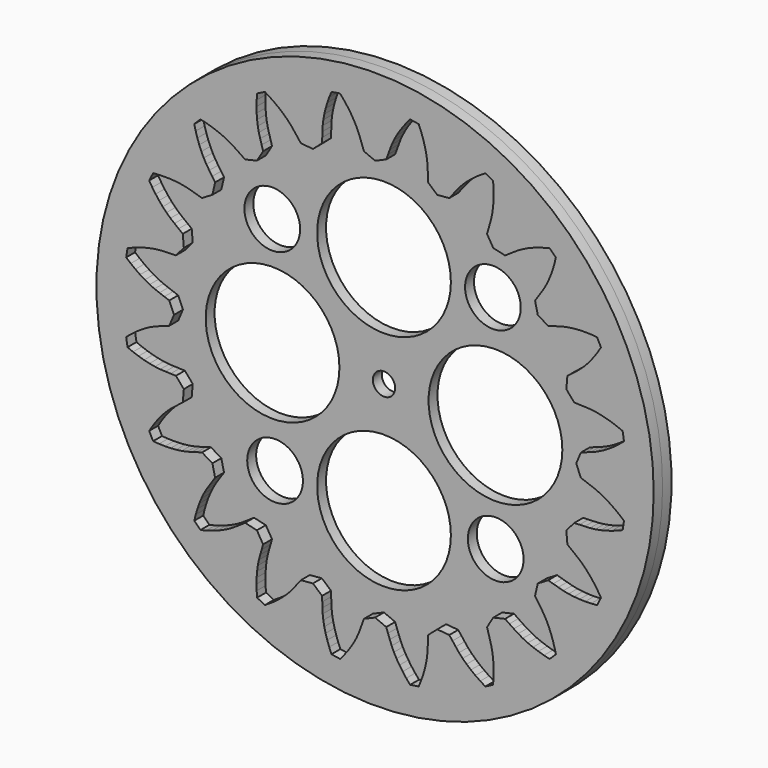
from build123d import *

# Parameters (mm, degrees)
F0_R     = 125
F1_DEPTH = 5
F2_R     = 125
F3_DEPTH = 5
F4_R     = 5
F5_DEPTH = 10.001
F6_R     = 30
F7_DEPTH = 5.001
F8_R     = 12.5
F9_DEPTH = 10.001


# Not quite as in the source:
# - ends of sketch curves that miss each other by under 0.0002 mm in the source are joined


with BuildPart() as f1:
    # F0 (on Front) → F1 (new body)
    with BuildSketch(Plane.XZ):
        Circle(F0_R)
        Polygon((13.9842229545, 109.6228580511), (15.7057802544, 111.6674669584), (19.5700724052, 111.0554232512), (20.5755500849, 108.5788944008), (21.4485215555, 106.1098402186), (22.1849061713, 103.653016947), (22.779065605, 101.2135667406), (23.2227934587, 98.7972702634), (23.5031701941, 96.4110969894), (23.6169992555, 94.0596036896), (23.6990010858, 91.7113680901), (23.7811743213, 89.3582248904), (27.8774327783, 85.7978872065), (33.2840906682, 86.2705394296), (34.7337131873, 88.1259711729), (36.1803125604, 89.9775337706), (37.6545753224, 91.8130253807), (39.2839627575, 93.57867791), (41.0632104221, 95.2726860912), (42.9777689252, 96.8970045446), (45.0176015427, 98.4517796161), (47.1751233459, 99.9361663084), (49.4442399292, 101.3487141929), (52.930256939, 99.572499698), (53.1212343584, 96.9064699183), (53.1884993548, 94.2884977338), (53.1296422324, 91.7243648109), (52.9408900729, 89.2207038275), (52.6162246508, 86.785549776), (52.1455100076, 84.4295237621), (51.5271162906, 82.1579453597), (50.8794594033, 79.8993005287), (50.2304503198, 77.6359355406), (53.0260192955, 72.9840387035), (58.3141129314, 71.7628090439), (60.2661460143, 73.0794722829), (62.2141084754, 74.3933890299), (64.1834143867, 75.6834724412), (66.2786700093, 76.8592005473), (68.4943121935, 77.9204791254), (70.8171076594, 78.8736672065), (73.2375549479, 79.7220024436), (75.7481813959, 80.4670274831), (78.3427412398, 81.1092455143), (81.1092595475, 78.3427262043), (80.4670415162, 75.7481663603), (79.7220164768, 73.2375409148), (78.8736802373, 70.8170926238), (77.9204921562, 68.4942981603), (76.8592125757, 66.2786559761), (75.6834844697, 64.1834003535), (74.3934000559, 62.2140944422), (73.0794833089, 60.2661329835), (71.76282007, 58.3140999006), (72.9840487272, 53.0260052624), (77.6359445619, 50.2304352843), (79.8993095501, 50.8794453702), (82.157954381, 51.5271002527), (84.4295327834, 52.1454939697), (86.7855597997, 52.6162076106), (89.2207138511, 52.9408730326), (91.7243748346, 53.1296251921), (94.2885077575, 53.1884813122), (96.9064799419, 53.1212163158), (99.5725097217, 52.930237894), (101.3487232143, 49.4442208842), (99.9361753297, 47.1751043009), (98.4517876351, 45.0175824977), (96.8970125636, 42.9777508825), (95.2726931078, 41.0631923794), (93.5786859289, 39.2839457173), (91.8130323973, 37.6545582821), (89.9775407871, 36.1802955202), (88.1259771871, 34.733696147), (86.2705454438, 33.2840746303), (85.7978922183, 27.8774167404), (89.3582299022, 23.7811572811), (91.7113720996, 23.6989840456), (94.0596076991, 23.6169812128), (96.4111020013, 23.5031521515), (98.7972742729, 23.222775416), (101.2135707501, 22.7790465599), (103.6530219588, 22.1848861239), (106.1098442281, 21.4485015081), (108.5788974079, 20.5755300376), (111.0554272607, 19.5700513555), (111.6674689632, 15.7057712331), (109.6228590534, 13.9842149355), (107.5444121621, 12.3909899788), (105.4353899991, 10.9314470105), (103.298940004, 9.6125364595), (101.1380251806, 8.4438479932), (98.9552807579, 7.4398267561), (96.7540526447, 6.6049172539), (94.5460876072, 5.8012836795), (92.3335086637, 4.9959711366), (90.2132399167, -7.0166e-06), (92.3335076613, -4.9959861721), (94.5460866048, -5.8012997174), (96.7540516423, -6.6049332918), (98.9552797555, -7.4398417917), (101.1380241782, -8.4438650335), (103.2989390016, -9.6125524974), (105.4353889967, -10.9314640507), (107.5444101574, -12.3910080214), (109.6228570487, -13.9842319758), (111.6674659561, -15.7057892758), (111.0554242535, -19.5700693981), (108.5788944008, -20.5755470778), (106.109841221, -21.4485185484), (103.6530179493, -22.1849031642), (101.213567743, -22.7790625979), (98.7972712658, -23.2227914539), (96.4110979918, -23.503167187), (94.0596036896, -23.6169962484), (91.7113680901, -23.6989980787), (89.3582258927, -23.7811713142), (85.7978872065, -27.8774307736), (86.270540432, -33.2840876611), (88.1259721753, -34.7337101802), (89.9775347729, -36.1803105557), (91.8130263831, -37.6545733177), (93.5786789124, -39.2839607528), (95.2726870936, -41.063207415), (96.897005547, -42.9777659181), (98.4517806185, -45.0175985356), (99.9361673108, -47.1751203388), (101.3487161977, -49.4442369221), (99.5725007004, -52.9302539319), (96.906471923, -53.1212313513), (94.2884987361, -53.1884963477), (91.7243668156, -53.1296402276), (89.2207058322, -52.9408880681), (86.7855517808, -52.6162216437), (84.4295247645, -52.1455080029), (82.157946362, -51.5271142859), (79.8993015311, -50.8794573986), (77.635936543, -50.2304483151), (72.9840407082, -53.0260172908), (71.7628110487, -58.314111929), (73.0794732852, -60.2661440096), (74.3933900322, -62.2141064707), (75.683474446, -64.1834123819), (76.8592015497, -66.2786680046), (77.9204811301, -68.4943101888), (78.8736682089, -70.8171056546), (79.7220044483, -73.2375529432), (80.4670294878, -75.7481793911), (81.1092475191, -78.3427392351), (78.342728209, -81.1092575428), (75.748168365, -80.4670395115), (73.2375429195, -79.722014472), (70.8170946286, -78.8736782326), (68.4943001651, -77.9204901514), (66.2786579809, -76.859210571), (64.1834023582, -75.6834824649), (62.214096447, -74.3933990536), (60.2661349882, -73.0794813042), (58.3141019053, -71.7628190676), (53.0260072671, -72.9840477248), (50.230437289, -77.6359435596), (50.8794473749, -79.8993085477), (51.5271032598, -82.1579533786), (52.1454969768, -84.429531781), (52.6162106177, -86.7855587974), (52.9408760397, -89.2207128488), (53.1296281992, -91.7243738322), (53.1884843193, -94.2885067551), (53.1212183205, -96.9064789396), (52.9302409011, -99.572507717), (49.4442238913, -101.3487222119), (47.175107308, -99.936173325), (45.0175855048, -98.4517866327), (42.9777528873, -96.8970115612), (41.0631953865, -95.2726921055), (39.283947722, -93.5786849266), (37.6545612893, -91.8130313949), (36.1802985273, -89.9775397848), (34.7336991541, -88.1259761848), (33.2840766351, -86.2705444415), (27.8774187451, -85.797891216), (23.7811592858, -89.3582288999), (23.6989860503, -91.7113710972), (23.61698422, -94.0596066967), (23.5031551586, -96.4111009989), (23.2227774208, -98.7972742729), (22.7790485647, -101.2135707501), (22.1848891311, -103.6530209564), (21.4485045152, -106.1098432257), (20.5755330447, -108.5788974079), (19.5700543626, -111.0554262583), (15.7057742402, -111.6674679608), (13.9842169403, -109.6228590534), (12.3909929859, -107.5444121621), (10.9314500176, -105.4353899991), (9.6125384642, -103.298940004), (8.4438510003, -101.1380251806), (7.4398287609, -98.9552807579), (6.604920261, -96.7540526447), (5.8012866866, -94.5460876072), (4.9959741437, -92.3335086637), (-5.0118e-06, -90.2132399167), (-4.9959841674, -92.3335086637), (-5.8012967103, -94.5460866048), (-6.6049302847, -96.7540516423), (-7.4398397869, -98.9552797555), (-8.4438620264, -101.1380241782), (-9.6125494903, -103.2989390016), (-10.9314610436, -105.4353889967), (-12.3910050143, -107.5444111598), (-13.9842289687, -109.6228570487), (-15.7057862687, -111.6674659561), (-19.570066391, -111.0554242535), (-20.5755450731, -108.5788954032), (-21.4485155413, -106.109841221), (-22.1849001571, -103.6530189517), (-22.7790595907, -101.213567743), (-23.2227884468, -98.7972712658), (-23.5031651823, -96.4110979918), (-23.6169942436, -94.059604692), (-23.698996074, -91.7113690925), (-23.7811693095, -89.3582258927), (-27.8774287688, -85.7978882088), (-33.2840856564, -86.2705414344), (-34.7337081754, -88.1259731776), (-36.1803075486, -89.9775357753), (-37.6545703106, -91.8130273854), (-39.2839577457, -93.5786809171), (-41.0632054102, -95.272688096), (-42.9777639133, -96.8970065494), (-45.0175955285, -98.4517816209), (-47.1751173317, -99.9361683131), (-49.4442349174, -101.3487172), (-52.9302519271, -99.5725027051), (-53.1212293466, -96.9064729254), (-53.188494343, -94.2885007409), (-53.1296382229, -91.724367818), (-52.940885061, -89.2207068346), (-52.616219639, -86.7855527831), (-52.1455059981, -84.4295257668), (-51.5271112788, -82.1579473644), (-50.8794553939, -79.8993025335), (-50.2304463104, -77.6359385477), (-53.026015286, -72.9840417106), (-58.3141099242, -71.762812051), (-60.2661420048, -73.07947529), (-62.2141044659, -74.393392037), (-64.1834103772, -75.6834764507), (-66.2786659998, -76.8592035544), (-68.494308184, -77.9204831349), (-70.8171036499, -78.8736702136), (-73.2375509384, -79.7220064531), (-75.7481773864, -80.4670314925), (-78.3427372303, -81.1092495238), (-81.109255538, -78.3427302138), (-80.4670375068, -75.7481703698), (-79.7220124673, -73.2375449242), (-78.8736762278, -70.8170976357), (-77.9204881467, -68.4943021698), (-76.8592085663, -66.2786599856), (-75.6834814626, -64.183404363), (-74.3933970488, -62.2140984517), (-73.0794803018, -60.266136993), (-71.7628170629, -58.31410391), (-72.9840457201, -53.0260092718), (-77.6359425572, -50.2304402961), (-79.899306543, -50.8794493796), (-82.1579513739, -51.5271052645), (-84.4295307787, -52.1454989815), (-86.7855567926, -52.6162126224), (-89.220710844, -52.9408780444), (-91.7243718275, -53.1296302039), (-94.2885047504, -53.188486324), (-96.9064769348, -53.1212213276), (-99.5725067146, -52.9302439082), (-101.3487212095, -49.4442258961), (-99.9361723226, -47.1751093127), (-98.4517856304, -45.0175875095), (-96.8970105589, -42.9777558944), (-95.2726911031, -41.0631973913), (-93.5786839242, -39.2839507291), (-91.8130303926, -37.654563294), (-89.9775387824, -36.180300532), (-88.1259761848, -34.7337011589), (-86.2705434391, -33.2840786398), (-85.7978902136, -27.8774217522), (-89.3582278975, -23.7811622929), (-91.7113710972, -23.698988055), (-94.0596066967, -23.6169862247), (-96.4110999965, -23.5031571633), (-98.7972732705, -23.2227804279), (-101.2135697477, -22.7790515718), (-103.6530199541, -22.1848921382), (-106.1098432257, -21.4485075223), (-108.5788964056, -20.5755360518), (-111.0554262583, -19.5700573697), (-111.6674679608, -15.7057772473), (-109.6228580511, -13.9842199474), (-107.5444121621, -12.390995993), (-105.4353899991, -10.9314520223), (-103.298940004, -9.6125414713), (-101.1380251806, -8.4438540074), (-98.9552807579, -7.439831768), (-96.7540526447, -6.6049222657), (-94.5460876072, -5.8012886914), (-92.3335086637, -4.9959761484), (-90.2132399167, 2.0047e-06), (-92.3335086637, 4.9959811602), (-94.5460866048, 5.8012937032), (-96.7540516423, 6.6049272776), (-98.9552807579, 7.4398367798), (-101.1380241782, 8.4438590193), (-103.2989390016, 9.6125474855), (-105.4353889967, 10.9314580365), (-107.5444111598, 12.3910020072), (-109.6228580511, 13.9842259616), (-111.6674669584, 15.7057832616), (-111.0554252559, 19.5700633839), (-108.5788954032, 20.575542066), (-106.1098422233, 21.4485125342), (-103.6530189517, 22.18489715), (-101.2135687453, 22.7790565836), (-98.7972722682, 23.2227854397), (-96.4110989942, 23.5031621752), (-94.0596056944, 23.6169912365), (-91.7113690925, 23.6989930669), (-89.3582268951, 23.7811673048), (-85.7978892112, 27.8774257617), (-86.2705414344, 33.2840836517), (-88.12597418, 34.7337061707), (-89.9775367777, 36.1803055439), (-91.8130283878, 37.6545683058), (-93.5786819195, 39.283955741), (-95.2726890983, 41.0632024031), (-96.8970075518, 42.9777609062), (-98.4517826233, 45.0175935237), (-99.9361693155, 47.1751153269), (-101.3487182024, 49.4442319103), (-99.5725037075, 52.93024892), (-96.9064749301, 53.1212263395), (-94.2885017433, 53.1884913359), (-91.7243688204, 53.1296352158), (-89.2207088393, 52.9408830563), (-86.7855547879, 52.6162176342), (-84.4295277716, 52.145502991), (-82.1579493691, 51.527109274), (-79.8993045382, 50.8794533891), (-77.6359395501, 50.2304443056), (-72.9840437153, 53.0260132813), (-71.7628140558, 58.3141079195), (-73.0794762924, 60.26614), (-74.3933940417, 62.2141024612), (-75.6834774531, 64.1834083725), (-76.8592055592, 66.2786639951), (-77.9204841372, 68.4943061793), (-78.8736722183, 70.8171016451), (-79.7220084578, 73.2375489337), (-80.4670334973, 75.7481743793), (-81.1092515286, 78.3427352256), (-78.3427322185, 81.1092535333), (-75.7481723745, 80.467035502), (-73.237546929, 79.7220104625), (-70.8170996404, 78.8736742231), (-68.4943041746, 77.920486142), (-66.2786619904, 76.8592075639), (-64.1834063677, 75.6834794578), (-62.2141004564, 74.3933950441), (-60.2661389977, 73.0794782971), (-58.3141059148, 71.7628150581), (-53.0260112766, 72.9840447177), (-50.2304423009, 77.6359405525), (-50.8794513844, 79.8993055406), (-51.5271072693, 82.1579503715), (-52.1455009863, 84.4295287739), (-52.6162146271, 86.7855557903), (-52.9408800492, 89.2207098417), (-53.129633211, 91.7243708251), (-53.1884893311, 94.288503748), (-53.1212243347, 96.9064759325), (-52.9302459129, 99.5725057122), (-49.4442289032, 101.3487202072), (-47.1751123198, 99.9361713202), (-45.0175905166, 98.451784628), (-42.9777589015, 96.8970085541), (-41.0632003984, 95.2726901007), (-39.2839527339, 93.5786829218), (-37.6545652987, 91.8130293902), (-36.1803025367, 89.97753778), (-34.7337031636, 88.1259751824), (-33.2840806446, 86.2705424367), (-27.877423757, 85.7978902136), (-23.7811642976, 89.3582278975), (-23.6989910621, 91.7113700949), (-23.6169892318, 94.0596056944), (-23.5031601704, 96.4110999965), (-23.222783435, 98.7972732705), (-22.7790545789, 101.2135687453), (-22.1848951453, 103.6530199541), (-21.4485095271, 106.1098422233), (-20.5755390589, 108.5788964056), (-19.5700603768, 111.0554252559), (-15.7057802544, 111.6674669584), (-13.9842229545, 109.6228580511), (-12.3909990001, 107.5444111598), (-10.9314550294, 105.4353889967), (-9.6125444784, 103.2989390016), (-8.4438570145, 101.1380251806), (-7.4398347751, 98.9552807579), (-6.6049252728, 96.7540516423), (-5.8012916985, 94.5460876072), (-4.9959791555, 92.3335086637), (0, 90.2132399167), (4.9959791555, 92.3335086637), (5.8012916985, 94.5460876072), (6.6049252728, 96.7540516423), (7.4398347751, 98.9552807579), (8.4438570145, 101.1380251806), (9.6125444784, 103.2989390016), (10.9314550294, 105.4353889967), (12.3909990001, 107.5444111598), align=None, mode=Mode.SUBTRACT)
    extrude(amount=F1_DEPTH)

    # F2 (on face) → F3 (join)
    with BuildSketch(Plane(origin=(0, 0, 0), x_dir=(-1, 0, 0), z_dir=(0, 1, 0))):
        Circle(F2_R)
        Polygon((-19.5700724052, 111.0554232512), (-15.7057802544, 111.6674669584), (-13.9842229545, 109.6228580511), (-12.3909990001, 107.5444111598), (-10.9314550294, 105.4353889967), (-9.6125444784, 103.2989390016), (-8.4438570145, 101.1380251806), (-7.4398347751, 98.9552807579), (-6.6049252728, 96.7540516423), (-5.8012916985, 94.5460876072), (-4.9959791555, 92.3335086637), (0, 90.2132399167), (4.9959791555, 92.3335086637), (5.8012916985, 94.5460876072), (6.6049252728, 96.7540516423), (7.4398347751, 98.9552807579), (8.4438570145, 101.1380251806), (9.6125444784, 103.2989390016), (10.9314550294, 105.4353889967), (12.3909990001, 107.5444111598), (13.9842229545, 109.6228580511), (15.7057802544, 111.6674669584), (19.5700603768, 111.0554252559), (20.5755390589, 108.5788964056), (21.4485095271, 106.1098422233), (22.1848951453, 103.6530199541), (22.7790545789, 101.2135687453), (23.222783435, 98.7972732705), (23.5031601704, 96.4110999965), (23.6169892318, 94.0596056944), (23.6989910621, 91.7113700949), (23.7811642976, 89.3582278975), (27.877423757, 85.7978902136), (33.2840806446, 86.2705424367), (34.7337031636, 88.1259751824), (36.1803025367, 89.97753778), (37.6545652987, 91.8130293902), (39.2839527339, 93.5786829218), (41.0632003984, 95.2726901007), (42.9777589015, 96.8970085541), (45.0175905166, 98.451784628), (47.1751123198, 99.9361713202), (49.4442289032, 101.3487202072), (52.9302459129, 99.5725057122), (53.1212243347, 96.9064759325), (53.1884893311, 94.288503748), (53.129633211, 91.7243708251), (52.9408800492, 89.2207098417), (52.6162146271, 86.7855557903), (52.1455009863, 84.4295287739), (51.5271072693, 82.1579503715), (50.8794513844, 79.8993055406), (50.2304423009, 77.6359405525), (53.0260112766, 72.9840447177), (58.3141059148, 71.7628150581), (60.2661389977, 73.0794782971), (62.2141004564, 74.3933950441), (64.1834063677, 75.6834794578), (66.2786619904, 76.8592075639), (68.4943041746, 77.920486142), (70.8170996404, 78.8736742231), (73.237546929, 79.7220104625), (75.7481723745, 80.467035502), (78.3427322185, 81.1092535333), (81.1092515286, 78.3427352256), (80.4670334973, 75.7481743793), (79.7220084578, 73.2375489337), (78.8736722183, 70.8171016451), (77.9204841372, 68.4943061793), (76.8592055592, 66.2786639951), (75.6834774531, 64.1834083725), (74.3933940417, 62.2141024612), (73.0794762924, 60.26614), (71.7628140558, 58.3141079195), (72.9840437153, 53.0260132813), (77.6359395501, 50.2304443056), (79.8993045382, 50.8794533891), (82.1579493691, 51.527109274), (84.4295277716, 52.145502991), (86.7855547879, 52.6162176342), (89.2207088393, 52.9408830563), (91.7243688204, 53.1296352158), (94.2885017433, 53.1884913359), (96.9064749301, 53.1212263395), (99.5725037075, 52.93024892), (101.3487182024, 49.4442319103), (99.9361693155, 47.1751153269), (98.4517826233, 45.0175935237), (96.8970075518, 42.9777609062), (95.2726890983, 41.0632024031), (93.5786819195, 39.283955741), (91.8130283878, 37.6545683058), (89.9775367777, 36.1803055439), (88.12597418, 34.7337061707), (86.2705414344, 33.2840836517), (85.7978892112, 27.8774257617), (89.3582268951, 23.7811673048), (91.7113690925, 23.6989930669), (94.0596056944, 23.6169912365), (96.4110989942, 23.5031621752), (98.7972722682, 23.2227854397), (101.2135687453, 22.7790565836), (103.6530189517, 22.18489715), (106.1098422233, 21.4485125342), (108.5788954032, 20.575542066), (111.0554252559, 19.5700633839), (111.6674669584, 15.7057832616), (109.6228580511, 13.9842259616), (107.5444111598, 12.3910020072), (105.4353889967, 10.9314580365), (103.2989390016, 9.6125474855), (101.1380241782, 8.4438590193), (98.9552807579, 7.4398367798), (96.7540516423, 6.6049272776), (94.5460866048, 5.8012937032), (92.3335086637, 4.9959811602), (90.2132399167, 2.0047e-06), (92.3335086637, -4.9959761484), (94.5460876072, -5.8012886914), (96.7540526447, -6.6049222657), (98.9552807579, -7.439831768), (101.1380251806, -8.4438540074), (103.298940004, -9.6125414713), (105.4353899991, -10.9314520223), (107.5444121621, -12.390995993), (109.6228580511, -13.9842199474), (111.6674679608, -15.7057772473), (111.0554262583, -19.5700573697), (108.5788964056, -20.5755360518), (106.1098432257, -21.4485075223), (103.6530199541, -22.1848921382), (101.2135697477, -22.7790515718), (98.7972732705, -23.2227804279), (96.4110999965, -23.5031571633), (94.0596066967, -23.6169862247), (91.7113710972, -23.698988055), (89.3582278975, -23.7811622929), (85.7978902136, -27.8774217522), (86.2705434391, -33.2840786398), (88.1259761848, -34.7337011589), (89.9775387824, -36.180300532), (91.8130303926, -37.654563294), (93.5786839242, -39.2839507291), (95.2726911031, -41.0631973913), (96.8970105589, -42.9777558944), (98.4517856304, -45.0175875095), (99.9361723226, -47.1751093127), (101.3487212095, -49.4442258961), (99.5725067146, -52.9302439082), (96.9064769348, -53.1212213276), (94.2885047504, -53.188486324), (91.7243718275, -53.1296302039), (89.220710844, -52.9408780444), (86.7855567926, -52.6162126224), (84.4295307787, -52.1454989815), (82.1579513739, -51.5271052645), (79.899306543, -50.8794493796), (77.6359425572, -50.2304402961), (72.9840457201, -53.0260092718), (71.7628170629, -58.31410391), (73.0794803018, -60.266136993), (74.3933970488, -62.2140984517), (75.6834814626, -64.183404363), (76.8592085663, -66.2786599856), (77.9204881467, -68.4943021698), (78.8736762278, -70.8170976357), (79.7220124673, -73.2375449242), (80.4670375068, -75.7481703698), (81.109255538, -78.3427302138), (78.3427372303, -81.1092495238), (75.7481773864, -80.4670314925), (73.2375509384, -79.7220064531), (70.8171036499, -78.8736702136), (68.494308184, -77.9204831349), (66.2786659998, -76.8592035544), (64.1834103772, -75.6834764507), (62.2141044659, -74.393392037), (60.2661420048, -73.07947529), (58.3141099242, -71.762812051), (53.026015286, -72.9840417106), (50.2304463104, -77.6359385477), (50.8794553939, -79.8993025335), (51.5271112788, -82.1579473644), (52.1455059981, -84.4295257668), (52.616219639, -86.7855527831), (52.940885061, -89.2207068346), (53.1296382229, -91.724367818), (53.188494343, -94.2885007409), (53.1212293466, -96.9064729254), (52.9302519271, -99.5725027051), (49.4442349174, -101.3487172), (47.1751173317, -99.9361683131), (45.0175955285, -98.4517816209), (42.9777639133, -96.8970065494), (41.0632054102, -95.272688096), (39.2839577457, -93.5786809171), (37.6545703106, -91.8130273854), (36.1803075486, -89.9775357753), (34.7337081754, -88.1259731776), (33.2840856564, -86.2705414344), (27.8774287688, -85.7978882088), (23.7811693095, -89.3582258927), (23.698996074, -91.7113690925), (23.6169942436, -94.059604692), (23.5031651823, -96.4110979918), (23.2227884468, -98.7972712658), (22.7790595907, -101.213567743), (22.1849001571, -103.6530189517), (21.4485155413, -106.109841221), (20.5755450731, -108.5788954032), (19.570066391, -111.0554242535), (15.7057862687, -111.6674659561), (13.9842289687, -109.6228570487), (12.3910050143, -107.5444111598), (10.9314610436, -105.4353889967), (9.6125494903, -103.2989390016), (8.4438620264, -101.1380241782), (7.4398397869, -98.9552797555), (6.6049302847, -96.7540516423), (5.8012967103, -94.5460866048), (4.9959841674, -92.3335086637), (5.0118e-06, -90.2132399167), (-4.9959741437, -92.3335086637), (-5.8012866866, -94.5460876072), (-6.604920261, -96.7540526447), (-7.4398287609, -98.9552807579), (-8.4438510003, -101.1380251806), (-9.6125384642, -103.298940004), (-10.9314500176, -105.4353899991), (-12.3909929859, -107.5444121621), (-13.9842169403, -109.6228590534), (-15.7057742402, -111.6674679608), (-19.5700543626, -111.0554262583), (-20.5755330447, -108.5788974079), (-21.4485045152, -106.1098432257), (-22.1848891311, -103.6530209564), (-22.7790485647, -101.2135707501), (-23.2227774208, -98.7972742729), (-23.5031551586, -96.4111009989), (-23.61698422, -94.0596066967), (-23.6989860503, -91.7113710972), (-23.7811592858, -89.3582288999), (-27.8774187451, -85.797891216), (-33.2840766351, -86.2705444415), (-34.7336991541, -88.1259761848), (-36.1802985273, -89.9775397848), (-37.6545612893, -91.8130313949), (-39.283947722, -93.5786849266), (-41.0631953865, -95.2726921055), (-42.9777528873, -96.8970115612), (-45.0175855048, -98.4517866327), (-47.175107308, -99.936173325), (-49.4442238913, -101.3487222119), (-52.9302409011, -99.572507717), (-53.1212183205, -96.9064789396), (-53.1884843193, -94.2885067551), (-53.1296281992, -91.7243738322), (-52.9408760397, -89.2207128488), (-52.6162106177, -86.7855587974), (-52.1454969768, -84.429531781), (-51.5271032598, -82.1579533786), (-50.8794473749, -79.8993085477), (-50.230437289, -77.6359435596), (-53.0260072671, -72.9840477248), (-58.3141019053, -71.7628190676), (-60.2661349882, -73.0794813042), (-62.214096447, -74.3933990536), (-64.1834023582, -75.6834824649), (-66.2786579809, -76.859210571), (-68.4943001651, -77.9204901514), (-70.8170946286, -78.8736782326), (-73.2375429195, -79.722014472), (-75.748168365, -80.4670395115), (-78.342728209, -81.1092575428), (-81.1092475191, -78.3427392351), (-80.4670294878, -75.7481793911), (-79.7220044483, -73.2375529432), (-78.8736682089, -70.8171056546), (-77.9204811301, -68.4943101888), (-76.8592015497, -66.2786680046), (-75.683474446, -64.1834123819), (-74.3933900322, -62.2141064707), (-73.0794732852, -60.2661440096), (-71.7628110487, -58.314111929), (-72.9840407082, -53.0260172908), (-77.635936543, -50.2304483151), (-79.8993015311, -50.8794573986), (-82.157946362, -51.5271142859), (-84.4295247645, -52.1455080029), (-86.7855517808, -52.6162216437), (-89.2207058322, -52.9408880681), (-91.7243668156, -53.1296402276), (-94.2884987361, -53.1884963477), (-96.906471923, -53.1212313513), (-99.5725007004, -52.9302539319), (-101.3487161977, -49.4442369221), (-99.9361673108, -47.1751203388), (-98.4517806185, -45.0175985356), (-96.897005547, -42.9777659181), (-95.2726870936, -41.063207415), (-93.5786789124, -39.2839607528), (-91.8130263831, -37.6545733177), (-89.9775347729, -36.1803105557), (-88.1259721753, -34.7337101802), (-86.270540432, -33.2840876611), (-85.7978872065, -27.8774307736), (-89.3582258927, -23.7811713142), (-91.7113680901, -23.6989980787), (-94.0596036896, -23.6169962484), (-96.4110979918, -23.503167187), (-98.7972712658, -23.2227914539), (-101.213567743, -22.7790625979), (-103.6530179493, -22.1849031642), (-106.109841221, -21.4485185484), (-108.5788944008, -20.5755470778), (-111.0554242535, -19.5700693981), (-111.6674659561, -15.7057892758), (-109.6228570487, -13.9842319758), (-107.5444101574, -12.3910080214), (-105.4353889967, -10.9314640507), (-103.2989390016, -9.6125524974), (-101.1380241782, -8.4438650335), (-98.9552797555, -7.4398417917), (-96.7540516423, -6.6049332918), (-94.5460866048, -5.8012997174), (-92.3335076613, -4.9959861721), (-90.2132399167, -7.0166e-06), (-92.3335086637, 4.9959711366), (-94.5460876072, 5.8012836795), (-96.7540526447, 6.6049172539), (-98.9552807579, 7.4398267561), (-101.1380251806, 8.4438479932), (-103.298940004, 9.6125364595), (-105.4353899991, 10.9314470105), (-107.5444121621, 12.3909899788), (-109.6228590534, 13.9842149355), (-111.6674689632, 15.7057712331), (-111.0554272607, 19.5700513555), (-108.5788974079, 20.5755300376), (-106.1098442281, 21.4485015081), (-103.6530219588, 22.1848861239), (-101.2135707501, 22.7790465599), (-98.7972742729, 23.222775416), (-96.4111020013, 23.5031521515), (-94.0596076991, 23.6169812128), (-91.7113720996, 23.6989840456), (-89.3582299022, 23.7811572811), (-85.7978922183, 27.8774167404), (-86.2705454438, 33.2840746303), (-88.1259771871, 34.733696147), (-89.9775407871, 36.1802955202), (-91.8130323973, 37.6545582821), (-93.5786859289, 39.2839457173), (-95.2726931078, 41.0631923794), (-96.8970125636, 42.9777508825), (-98.4517876351, 45.0175824977), (-99.9361753297, 47.1751043009), (-101.3487232143, 49.4442208842), (-99.5725097217, 52.930237894), (-96.9064799419, 53.1212163158), (-94.2885077575, 53.1884813122), (-91.7243748346, 53.1296251921), (-89.2207138511, 52.9408730326), (-86.7855597997, 52.6162076106), (-84.4295327834, 52.1454939697), (-82.157954381, 51.5271002527), (-79.8993095501, 50.8794453702), (-77.6359445619, 50.2304352843), (-72.9840487272, 53.0260052624), (-71.76282007, 58.3140999006), (-73.0794833089, 60.2661329835), (-74.3934000559, 62.2140944422), (-75.6834844697, 64.1834003535), (-76.8592125757, 66.2786559761), (-77.9204921562, 68.4942981603), (-78.8736802373, 70.8170926238), (-79.7220164768, 73.2375409148), (-80.4670415162, 75.7481663603), (-81.1092595475, 78.3427262043), (-78.3427412398, 81.1092455143), (-75.7481813959, 80.4670274831), (-73.2375549479, 79.7220024436), (-70.8171076594, 78.8736672065), (-68.4943121935, 77.9204791254), (-66.2786700093, 76.8592005473), (-64.1834143867, 75.6834724412), (-62.2141084754, 74.3933890299), (-60.2661460143, 73.0794722829), (-58.3141129314, 71.7628090439), (-53.0260192955, 72.9840387035), (-50.2304503198, 77.6359355406), (-50.8794594033, 79.8993005287), (-51.5271162906, 82.1579453597), (-52.1455100076, 84.4295237621), (-52.6162246508, 86.785549776), (-52.9408900729, 89.2207038275), (-53.1296422324, 91.7243648109), (-53.1884993548, 94.2884977338), (-53.1212343584, 96.9064699183), (-52.930256939, 99.572499698), (-49.4442399292, 101.3487141929), (-47.1751233459, 99.9361663084), (-45.0176015427, 98.4517796161), (-42.9777689252, 96.8970045446), (-41.0632104221, 95.2726860912), (-39.2839627575, 93.57867791), (-37.6545753224, 91.8130253807), (-36.1803125604, 89.9775337706), (-34.7337131873, 88.1259711729), (-33.2840906682, 86.2705394296), (-27.8774327783, 85.7978872065), (-23.7811743213, 89.3582248904), (-23.6990010858, 91.7113680901), (-23.6169992555, 94.0596036896), (-23.5031701941, 96.4110969894), (-23.2227934587, 98.7972702634), (-22.779065605, 101.2135667406), (-22.1849061713, 103.653016947), (-21.4485215555, 106.1098402186), (-20.5755500849, 108.5788944008), align=None, mode=Mode.SUBTRACT)
        Polygon((-13.9842229545, 109.6228580511), (-15.7057802544, 111.6674669584), (-19.5700724052, 111.0554232512), (-20.5755500849, 108.5788944008), (-21.4485215555, 106.1098402186), (-22.1849061713, 103.653016947), (-22.779065605, 101.2135667406), (-23.2227934587, 98.7972702634), (-23.5031701941, 96.4110969894), (-23.6169992555, 94.0596036896), (-23.6990010858, 91.7113680901), (-23.7811743213, 89.3582248904), (-27.8774327783, 85.7978872065), (-33.2840906682, 86.2705394296), (-34.7337131873, 88.1259711729), (-36.1803125604, 89.9775337706), (-37.6545753224, 91.8130253807), (-39.2839627575, 93.57867791), (-41.0632104221, 95.2726860912), (-42.9777689252, 96.8970045446), (-45.0176015427, 98.4517796161), (-47.1751233459, 99.9361663084), (-49.4442399292, 101.3487141929), (-52.930256939, 99.572499698), (-53.1212343584, 96.9064699183), (-53.1884993548, 94.2884977338), (-53.1296422324, 91.7243648109), (-52.9408900729, 89.2207038275), (-52.6162246508, 86.785549776), (-52.1455100076, 84.4295237621), (-51.5271162906, 82.1579453597), (-50.8794594033, 79.8993005287), (-50.2304503198, 77.6359355406), (-53.0260192955, 72.9840387035), (-58.3141129314, 71.7628090439), (-60.2661460143, 73.0794722829), (-62.2141084754, 74.3933890299), (-64.1834143867, 75.6834724412), (-66.2786700093, 76.8592005473), (-68.4943121935, 77.9204791254), (-70.8171076594, 78.8736672065), (-73.2375549479, 79.7220024436), (-75.7481813959, 80.4670274831), (-78.3427412398, 81.1092455143), (-81.1092595475, 78.3427262043), (-80.4670415162, 75.7481663603), (-79.7220164768, 73.2375409148), (-78.8736802373, 70.8170926238), (-77.9204921562, 68.4942981603), (-76.8592125757, 66.2786559761), (-75.6834844697, 64.1834003535), (-74.3934000559, 62.2140944422), (-73.0794833089, 60.2661329835), (-71.76282007, 58.3140999006), (-72.9840487272, 53.0260052624), (-77.6359445619, 50.2304352843), (-79.8993095501, 50.8794453702), (-82.157954381, 51.5271002527), (-84.4295327834, 52.1454939697), (-86.7855597997, 52.6162076106), (-89.2207138511, 52.9408730326), (-91.7243748346, 53.1296251921), (-94.2885077575, 53.1884813122), (-96.9064799419, 53.1212163158), (-99.5725097217, 52.930237894), (-101.3487232143, 49.4442208842), (-99.9361753297, 47.1751043009), (-98.4517876351, 45.0175824977), (-96.8970125636, 42.9777508825), (-95.2726931078, 41.0631923794), (-93.5786859289, 39.2839457173), (-91.8130323973, 37.6545582821), (-89.9775407871, 36.1802955202), (-88.1259771871, 34.733696147), (-86.2705454438, 33.2840746303), (-85.7978922183, 27.8774167404), (-89.3582299022, 23.7811572811), (-91.7113720996, 23.6989840456), (-94.0596076991, 23.6169812128), (-96.4111020013, 23.5031521515), (-98.7972742729, 23.222775416), (-101.2135707501, 22.7790465599), (-103.6530219588, 22.1848861239), (-106.1098442281, 21.4485015081), (-108.5788974079, 20.5755300376), (-111.0554272607, 19.5700513555), (-111.6674689632, 15.7057712331), (-109.6228590534, 13.9842149355), (-107.5444121621, 12.3909899788), (-105.4353899991, 10.9314470105), (-103.298940004, 9.6125364595), (-101.1380251806, 8.4438479932), (-98.9552807579, 7.4398267561), (-96.7540526447, 6.6049172539), (-94.5460876072, 5.8012836795), (-92.3335086637, 4.9959711366), (-90.2132399167, -7.0166e-06), (-92.3335076613, -4.9959861721), (-94.5460866048, -5.8012997174), (-96.7540516423, -6.6049332918), (-98.9552797555, -7.4398417917), (-101.1380241782, -8.4438650335), (-103.2989390016, -9.6125524974), (-105.4353889967, -10.9314640507), (-107.5444101574, -12.3910080214), (-109.6228570487, -13.9842319758), (-111.6674659561, -15.7057892758), (-111.0554242535, -19.5700693981), (-108.5788944008, -20.5755470778), (-106.109841221, -21.4485185484), (-103.6530179493, -22.1849031642), (-101.213567743, -22.7790625979), (-98.7972712658, -23.2227914539), (-96.4110979918, -23.503167187), (-94.0596036896, -23.6169962484), (-91.7113680901, -23.6989980787), (-89.3582258927, -23.7811713142), (-85.7978872065, -27.8774307736), (-86.270540432, -33.2840876611), (-88.1259721753, -34.7337101802), (-89.9775347729, -36.1803105557), (-91.8130263831, -37.6545733177), (-93.5786789124, -39.2839607528), (-95.2726870936, -41.063207415), (-96.897005547, -42.9777659181), (-98.4517806185, -45.0175985356), (-99.9361673108, -47.1751203388), (-101.3487161977, -49.4442369221), (-99.5725007004, -52.9302539319), (-96.906471923, -53.1212313513), (-94.2884987361, -53.1884963477), (-91.7243668156, -53.1296402276), (-89.2207058322, -52.9408880681), (-86.7855517808, -52.6162216437), (-84.4295247645, -52.1455080029), (-82.157946362, -51.5271142859), (-79.8993015311, -50.8794573986), (-77.635936543, -50.2304483151), (-72.9840407082, -53.0260172908), (-71.7628110487, -58.314111929), (-73.0794732852, -60.2661440096), (-74.3933900322, -62.2141064707), (-75.683474446, -64.1834123819), (-76.8592015497, -66.2786680046), (-77.9204811301, -68.4943101888), (-78.8736682089, -70.8171056546), (-79.7220044483, -73.2375529432), (-80.4670294878, -75.7481793911), (-81.1092475191, -78.3427392351), (-78.342728209, -81.1092575428), (-75.748168365, -80.4670395115), (-73.2375429195, -79.722014472), (-70.8170946286, -78.8736782326), (-68.4943001651, -77.9204901514), (-66.2786579809, -76.859210571), (-64.1834023582, -75.6834824649), (-62.214096447, -74.3933990536), (-60.2661349882, -73.0794813042), (-58.3141019053, -71.7628190676), (-53.0260072671, -72.9840477248), (-50.230437289, -77.6359435596), (-50.8794473749, -79.8993085477), (-51.5271032598, -82.1579533786), (-52.1454969768, -84.429531781), (-52.6162106177, -86.7855587974), (-52.9408760397, -89.2207128488), (-53.1296281992, -91.7243738322), (-53.1884843193, -94.2885067551), (-53.1212183205, -96.9064789396), (-52.9302409011, -99.572507717), (-49.4442238913, -101.3487222119), (-47.175107308, -99.936173325), (-45.0175855048, -98.4517866327), (-42.9777528873, -96.8970115612), (-41.0631953865, -95.2726921055), (-39.283947722, -93.5786849266), (-37.6545612893, -91.8130313949), (-36.1802985273, -89.9775397848), (-34.7336991541, -88.1259761848), (-33.2840766351, -86.2705444415), (-27.8774187451, -85.797891216), (-23.7811592858, -89.3582288999), (-23.6989860503, -91.7113710972), (-23.61698422, -94.0596066967), (-23.5031551586, -96.4111009989), (-23.2227774208, -98.7972742729), (-22.7790485647, -101.2135707501), (-22.1848891311, -103.6530209564), (-21.4485045152, -106.1098432257), (-20.5755330447, -108.5788974079), (-19.5700543626, -111.0554262583), (-15.7057742402, -111.6674679608), (-13.9842169403, -109.6228590534), (-12.3909929859, -107.5444121621), (-10.9314500176, -105.4353899991), (-9.6125384642, -103.298940004), (-8.4438510003, -101.1380251806), (-7.4398287609, -98.9552807579), (-6.604920261, -96.7540526447), (-5.8012866866, -94.5460876072), (-4.9959741437, -92.3335086637), (5.0118e-06, -90.2132399167), (4.9959841674, -92.3335086637), (5.8012967103, -94.5460866048), (6.6049302847, -96.7540516423), (7.4398397869, -98.9552797555), (8.4438620264, -101.1380241782), (9.6125494903, -103.2989390016), (10.9314610436, -105.4353889967), (12.3910050143, -107.5444111598), (13.9842289687, -109.6228570487), (15.7057862687, -111.6674659561), (19.570066391, -111.0554242535), (20.5755450731, -108.5788954032), (21.4485155413, -106.109841221), (22.1849001571, -103.6530189517), (22.7790595907, -101.213567743), (23.2227884468, -98.7972712658), (23.5031651823, -96.4110979918), (23.6169942436, -94.059604692), (23.698996074, -91.7113690925), (23.7811693095, -89.3582258927), (27.8774287688, -85.7978882088), (33.2840856564, -86.2705414344), (34.7337081754, -88.1259731776), (36.1803075486, -89.9775357753), (37.6545703106, -91.8130273854), (39.2839577457, -93.5786809171), (41.0632054102, -95.272688096), (42.9777639133, -96.8970065494), (45.0175955285, -98.4517816209), (47.1751173317, -99.9361683131), (49.4442349174, -101.3487172), (52.9302519271, -99.5725027051), (53.1212293466, -96.9064729254), (53.188494343, -94.2885007409), (53.1296382229, -91.724367818), (52.940885061, -89.2207068346), (52.616219639, -86.7855527831), (52.1455059981, -84.4295257668), (51.5271112788, -82.1579473644), (50.8794553939, -79.8993025335), (50.2304463104, -77.6359385477), (53.026015286, -72.9840417106), (58.3141099242, -71.762812051), (60.2661420048, -73.07947529), (62.2141044659, -74.393392037), (64.1834103772, -75.6834764507), (66.2786659998, -76.8592035544), (68.494308184, -77.9204831349), (70.8171036499, -78.8736702136), (73.2375509384, -79.7220064531), (75.7481773864, -80.4670314925), (78.3427372303, -81.1092495238), (81.109255538, -78.3427302138), (80.4670375068, -75.7481703698), (79.7220124673, -73.2375449242), (78.8736762278, -70.8170976357), (77.9204881467, -68.4943021698), (76.8592085663, -66.2786599856), (75.6834814626, -64.183404363), (74.3933970488, -62.2140984517), (73.0794803018, -60.266136993), (71.7628170629, -58.31410391), (72.9840457201, -53.0260092718), (77.6359425572, -50.2304402961), (79.899306543, -50.8794493796), (82.1579513739, -51.5271052645), (84.4295307787, -52.1454989815), (86.7855567926, -52.6162126224), (89.220710844, -52.9408780444), (91.7243718275, -53.1296302039), (94.2885047504, -53.188486324), (96.9064769348, -53.1212213276), (99.5725067146, -52.9302439082), (101.3487212095, -49.4442258961), (99.9361723226, -47.1751093127), (98.4517856304, -45.0175875095), (96.8970105589, -42.9777558944), (95.2726911031, -41.0631973913), (93.5786839242, -39.2839507291), (91.8130303926, -37.654563294), (89.9775387824, -36.180300532), (88.1259761848, -34.7337011589), (86.2705434391, -33.2840786398), (85.7978902136, -27.8774217522), (89.3582278975, -23.7811622929), (91.7113710972, -23.698988055), (94.0596066967, -23.6169862247), (96.4110999965, -23.5031571633), (98.7972732705, -23.2227804279), (101.2135697477, -22.7790515718), (103.6530199541, -22.1848921382), (106.1098432257, -21.4485075223), (108.5788964056, -20.5755360518), (111.0554262583, -19.5700573697), (111.6674679608, -15.7057772473), (109.6228580511, -13.9842199474), (107.5444121621, -12.390995993), (105.4353899991, -10.9314520223), (103.298940004, -9.6125414713), (101.1380251806, -8.4438540074), (98.9552807579, -7.439831768), (96.7540526447, -6.6049222657), (94.5460876072, -5.8012886914), (92.3335086637, -4.9959761484), (90.2132399167, 2.0047e-06), (92.3335086637, 4.9959811602), (94.5460866048, 5.8012937032), (96.7540516423, 6.6049272776), (98.9552807579, 7.4398367798), (101.1380241782, 8.4438590193), (103.2989390016, 9.6125474855), (105.4353889967, 10.9314580365), (107.5444111598, 12.3910020072), (109.6228580511, 13.9842259616), (111.6674669584, 15.7057832616), (111.0554252559, 19.5700633839), (108.5788954032, 20.575542066), (106.1098422233, 21.4485125342), (103.6530189517, 22.18489715), (101.2135687453, 22.7790565836), (98.7972722682, 23.2227854397), (96.4110989942, 23.5031621752), (94.0596056944, 23.6169912365), (91.7113690925, 23.6989930669), (89.3582268951, 23.7811673048), (85.7978892112, 27.8774257617), (86.2705414344, 33.2840836517), (88.12597418, 34.7337061707), (89.9775367777, 36.1803055439), (91.8130283878, 37.6545683058), (93.5786819195, 39.283955741), (95.2726890983, 41.0632024031), (96.8970075518, 42.9777609062), (98.4517826233, 45.0175935237), (99.9361693155, 47.1751153269), (101.3487182024, 49.4442319103), (99.5725037075, 52.93024892), (96.9064749301, 53.1212263395), (94.2885017433, 53.1884913359), (91.7243688204, 53.1296352158), (89.2207088393, 52.9408830563), (86.7855547879, 52.6162176342), (84.4295277716, 52.145502991), (82.1579493691, 51.527109274), (79.8993045382, 50.8794533891), (77.6359395501, 50.2304443056), (72.9840437153, 53.0260132813), (71.7628140558, 58.3141079195), (73.0794762924, 60.26614), (74.3933940417, 62.2141024612), (75.6834774531, 64.1834083725), (76.8592055592, 66.2786639951), (77.9204841372, 68.4943061793), (78.8736722183, 70.8171016451), (79.7220084578, 73.2375489337), (80.4670334973, 75.7481743793), (81.1092515286, 78.3427352256), (78.3427322185, 81.1092535333), (75.7481723745, 80.467035502), (73.237546929, 79.7220104625), (70.8170996404, 78.8736742231), (68.4943041746, 77.920486142), (66.2786619904, 76.8592075639), (64.1834063677, 75.6834794578), (62.2141004564, 74.3933950441), (60.2661389977, 73.0794782971), (58.3141059148, 71.7628150581), (53.0260112766, 72.9840447177), (50.2304423009, 77.6359405525), (50.8794513844, 79.8993055406), (51.5271072693, 82.1579503715), (52.1455009863, 84.4295287739), (52.6162146271, 86.7855557903), (52.9408800492, 89.2207098417), (53.129633211, 91.7243708251), (53.1884893311, 94.288503748), (53.1212243347, 96.9064759325), (52.9302459129, 99.5725057122), (49.4442289032, 101.3487202072), (47.1751123198, 99.9361713202), (45.0175905166, 98.451784628), (42.9777589015, 96.8970085541), (41.0632003984, 95.2726901007), (39.2839527339, 93.5786829218), (37.6545652987, 91.8130293902), (36.1803025367, 89.97753778), (34.7337031636, 88.1259751824), (33.2840806446, 86.2705424367), (27.877423757, 85.7978902136), (23.7811642976, 89.3582278975), (23.6989910621, 91.7113700949), (23.6169892318, 94.0596056944), (23.5031601704, 96.4110999965), (23.222783435, 98.7972732705), (22.7790545789, 101.2135687453), (22.1848951453, 103.6530199541), (21.4485095271, 106.1098422233), (20.5755390589, 108.5788964056), (19.5700603768, 111.0554252559), (15.7057802544, 111.6674669584), (13.9842229545, 109.6228580511), (12.3909990001, 107.5444111598), (10.9314550294, 105.4353889967), (9.6125444784, 103.2989390016), (8.4438570145, 101.1380251806), (7.4398347751, 98.9552807579), (6.6049252728, 96.7540516423), (5.8012916985, 94.5460876072), (4.9959791555, 92.3335086637), (0, 90.2132399167), (-4.9959791555, 92.3335086637), (-5.8012916985, 94.5460876072), (-6.6049252728, 96.7540516423), (-7.4398347751, 98.9552807579), (-8.4438570145, 101.1380251806), (-9.6125444784, 103.2989390016), (-10.9314550294, 105.4353889967), (-12.3909990001, 107.5444111598), align=None)
    extrude(amount=F3_DEPTH)

    # F4 (on face) → F5 (cut, through all)
    with BuildSketch(Plane(origin=(0, 5, 0), x_dir=(-1, 0, 0), z_dir=(0, 1, 0))):
        Circle(F4_R)
    extrude(amount=-F5_DEPTH, mode=Mode.SUBTRACT)

    # F6 (on face) → F7 (cut, through all)
    with BuildSketch(Plane.XZ):
        with Locations((50, 0)):
            Circle(F6_R)
        with Locations((0, 50)):
            Circle(F6_R)
        with Locations((-50, 0)):
            Circle(F6_R)
        with Locations((0, -50)):
            Circle(F6_R)
    extrude(amount=-F7_DEPTH, mode=Mode.SUBTRACT)

    # F8 (on face) → F9 (cut, through all)
    with BuildSketch(Plane(origin=(0, 5, 0), x_dir=(-1, 0, 0), z_dir=(0, 1, 0))):
        with Locations((-50.1177805749, -48.8692957822)):
            Circle(F8_R)
        with Locations((48.8692957822, -50.1177805749)):
            Circle(F8_R)
        with Locations((50.1177805749, 48.8692957822)):
            Circle(F8_R)
        with Locations((-48.8692957822, 50.1177805749)):
            Circle(F8_R)
    extrude(amount=-F9_DEPTH, mode=Mode.SUBTRACT)


solid = f1.part
